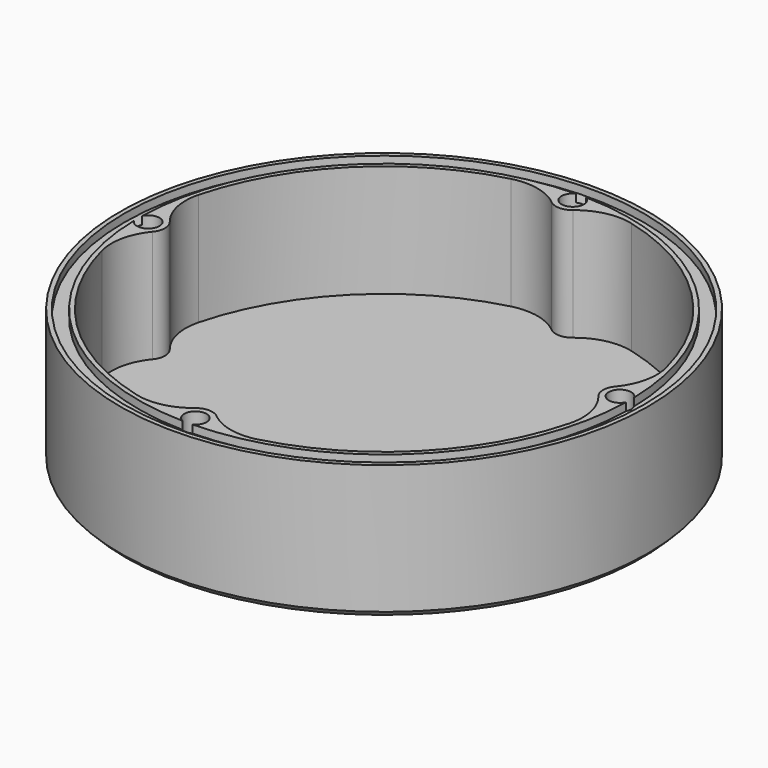
from build123d import *

# Parameters (mm, degrees)
F0_R      = 23.5
F1_DEPTH  = 12
F2_T      = -2
F3_SIZE   = 0.5
F4_R      = 1.5
F5_DEPTH  = 10
F6_R      = 5
F7_R      = 1
F8_DEPTH  = 12.001
F9_R      = 23.1
F9_R_2    = 21.9
F10_DEPTH = 0.7


# Not quite as in the source:
# - a fillet or chamfer that OpenCascade refuses, or shapes differently, is made with other operations: its cross-section is extruded or revolved along the edge and cut away or added


with BuildPart() as f1:
    # F0 (on Top) → F1 (new body)
    with BuildSketch(Plane.XY):
        Circle(F0_R)
    extrude(amount=F1_DEPTH)

    # F2
    f2_openings = [f1.faces().sort_by_distance(p)[0] for p in [
        (0, 0, 12),
    ]]
    offset(amount=F2_T, openings=f2_openings)

    # F3
    f3_edges = [f1.edges().sort_by_distance(p)[0] for p in [
        (-23.5, 0, 0),
    ]]
    chamfer(f3_edges, length=F3_SIZE)

    # F4 (on face) → F5 (join, through all)
    with BuildSketch(Plane.XY.offset(2)):
        with Locations((0, -21)):
            Circle(F4_R)
        with Locations((21, 0)):
            Circle(F4_R)
        with Locations((0, 21)):
            Circle(F4_R)
        with Locations((-21, 0)):
            Circle(F4_R)
    extrude(amount=F5_DEPTH)

    # F6
    f6_edges = [f1.edges().sort_by_distance(p)[0] for p in [
        (-21.452381, 1.430158, 7),
        (-21.452381, -1.430158, 7),
        (-1.430158, 21.452381, 7),
        (1.430158, 21.452381, 7),
        (21.452381, -1.430158, 7),
        (21.452381, 1.430158, 7),
        (-1.430158, -21.452381, 7),
        (1.430158, -21.452381, 7),
    ]]
    fillet(f6_edges, radius=F6_R)

    # F7 (on face) → F8 (cut, through all)
    with BuildSketch(Plane.XY.offset(12)):
        with Locations((0, -21)):
            Circle(F7_R)
        with Locations((21, 0)):
            Circle(F7_R)
        with Locations((0, 21)):
            Circle(F7_R)
        with Locations((-21, 0)):
            Circle(F7_R)
    extrude(amount=-F8_DEPTH, mode=Mode.SUBTRACT)

    # F9 (on face) → F10 (cut)
    with BuildSketch(Plane.XY.offset(12)):
        Circle(F9_R)
        Circle(F9_R_2, mode=Mode.SUBTRACT)
    extrude(amount=-F10_DEPTH, mode=Mode.SUBTRACT)

    # F11: chamfer of 1.2 on 4 edges, made by hand

    # F11_s1 → F11_t2 (revolve, cut)
    with BuildSketch(Plane.XZ.offset(-21)):
        Polygon((2.2, 0), (1, 1.2), (1, 0), align=None)
    revolve(axis=Axis((0, 21, 0), (0, 0, 1)), mode=Mode.SUBTRACT)

    # F11_s3 → F11_t4 (revolve, cut)
    with BuildSketch(Plane.XZ):
        Polygon((23.2, 0), (22, 1.2), (22, 0), align=None)
    revolve(axis=Axis((21, 0, 0), (0, 0, 1)), mode=Mode.SUBTRACT)

    # F11_s5 → F11_t6 (revolve, cut)
    with BuildSketch(Plane.XZ.offset(21)):
        Polygon((2.2, 0), (1, 1.2), (1, 0), align=None)
    revolve(axis=Axis((0, -21, 0), (0, 0, 1)), mode=Mode.SUBTRACT)

    # F11_s7 → F11_t8 (revolve, cut)
    with BuildSketch(Plane.XZ):
        Polygon((-18.8, 0), (-20, 1.2), (-20, 0), align=None)
    revolve(axis=Axis((-21, 0, 0), (0, 0, 1)), mode=Mode.SUBTRACT)


solid = f1.part
